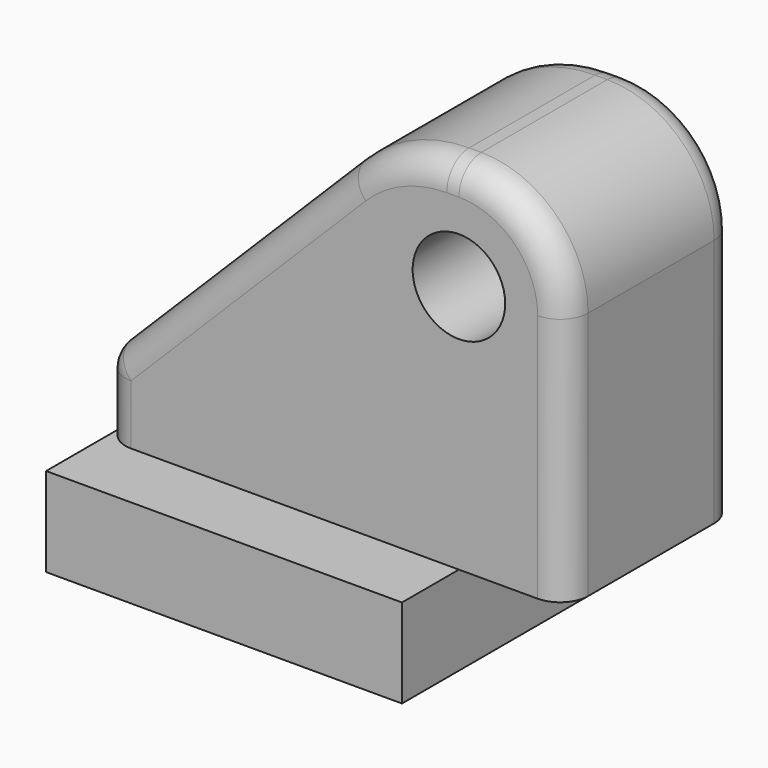
from build123d import *

# Parameters (mm, degrees)
F0_W     = 25.4
F0_H     = 25.4
F1_DEPTH = 6.35
F2_W     = 25.4
F2_H     = 15.24
F2_W_2   = 7.62
F3_DEPTH = 25.4
F4_R     = 7.62
F5_SIZE  = 20.32
F6_R     = 10.16
F7_R     = 3.302
F8_DEPTH = 20.321
F9_R     = 2


with BuildPart() as f1:
    # F0 (on Top) → F1 (new body)
    with BuildSketch(Plane.XY):
        Rectangle(F0_W, F0_H)
    extrude(amount=F1_DEPTH)

    # F2 (on face) → F3 (join)
    with BuildSketch(Plane.XY.offset(6.35)):
        Rectangle(F2_W, F2_H)
        with Locations((16.51, 0)):
            Rectangle(F2_W_2, F2_H)
    extrude(amount=F3_DEPTH)

    # F4
    f4_edges = [f1.edges().sort_by_distance(p)[0] for p in [
        (20.32, 0, 31.75),
    ]]
    fillet(f4_edges, radius=F4_R)

    # F5
    f5_edges = [f1.edges().sort_by_distance(p)[0] for p in [
        (-12.7, 0, 31.75),
    ]]
    chamfer(f5_edges, length=F5_SIZE)

    # F6
    f6_edges = [f1.edges().sort_by_distance(p)[0] for p in [
        (7.62, 0, 31.75),
    ]]
    fillet(f6_edges, radius=F6_R)

    # F7 (on face) → F8 (cut, through all)
    with BuildSketch(Plane.XZ.offset(7.62)):
        with Locations((12.7, 24.13)):
            Circle(F7_R)
    extrude(amount=-F8_DEPTH, mode=Mode.SUBTRACT)

    # F9
    f9_edges = [f1.edges().sort_by_distance(p)[0] for p in [
        (-4.027898, -7.62, 20.102102),
        (-4.027898, 7.62, 20.102102),
        (-12.7, 0, 11.43),
        (-12.7, -7.62, 8.89),
        (-12.7, 7.62, 8.89),
        (12.264205, -7.62, 31.75),
        (7.940346, -7.62, 30.976616),
        (18.088154, -7.62, 29.518154),
        (20.32, -7.62, 15.24),
        (12.264205, 7.62, 31.75),
        (7.940346, 7.62, 30.976616),
        (18.088154, 7.62, 29.518154),
        (20.32, 7.62, 15.24),
    ]]
    fillet(f9_edges, radius=F9_R)


solid = f1.part
